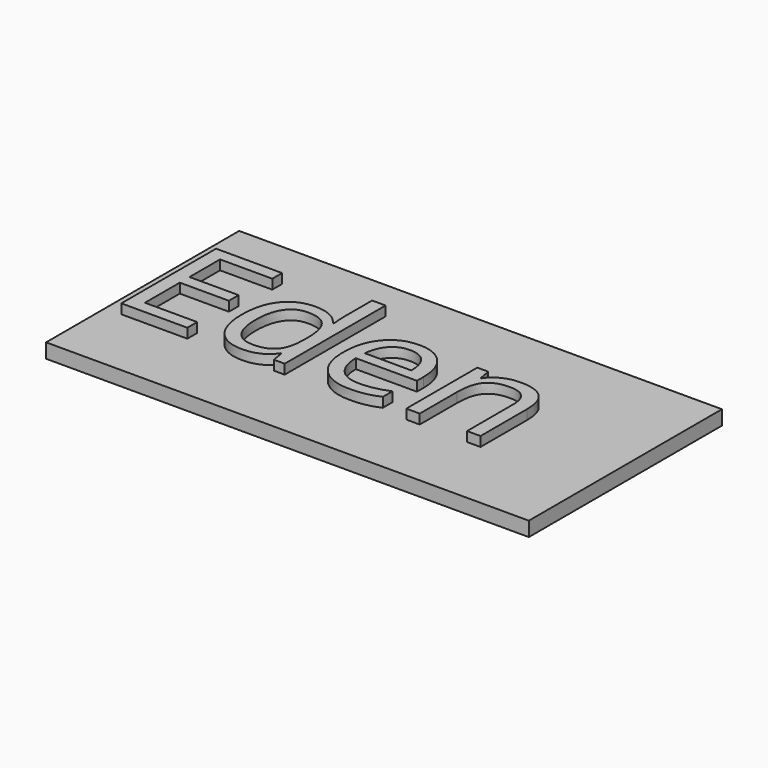
from build123d import *

# Parameters (mm, degrees)
F0_W         = 100
F0_H         = 50
F1_DEPTH     = 3
F2_TEXT_SIZE = 34.3624161074
F3_DEPTH     = 2


# Not quite as in the source:
# - Text() gives the source's letters only with a copy of the font that has no kerning and outlines rounded to 1/6400 em; it was checked with that copy


with BuildPart() as f1:
    # F0 (on Top) → F1 (new body)
    with BuildSketch(Plane.XY):
        with Locations((50, 25)):
            Rectangle(F0_W, F0_H)
    extrude(amount=F1_DEPTH)

    # F2 (on face) → F3 (join)
    with BuildSketch(Plane.XY.offset(3)):
        with Locations((0, 15.2717930165)):
            Text('Eden', F2_TEXT_SIZE, font='Open Sans', text_align=(TextAlign.LEFT, TextAlign.BOTTOM))
    extrude(amount=F3_DEPTH)


solid = f1.part
